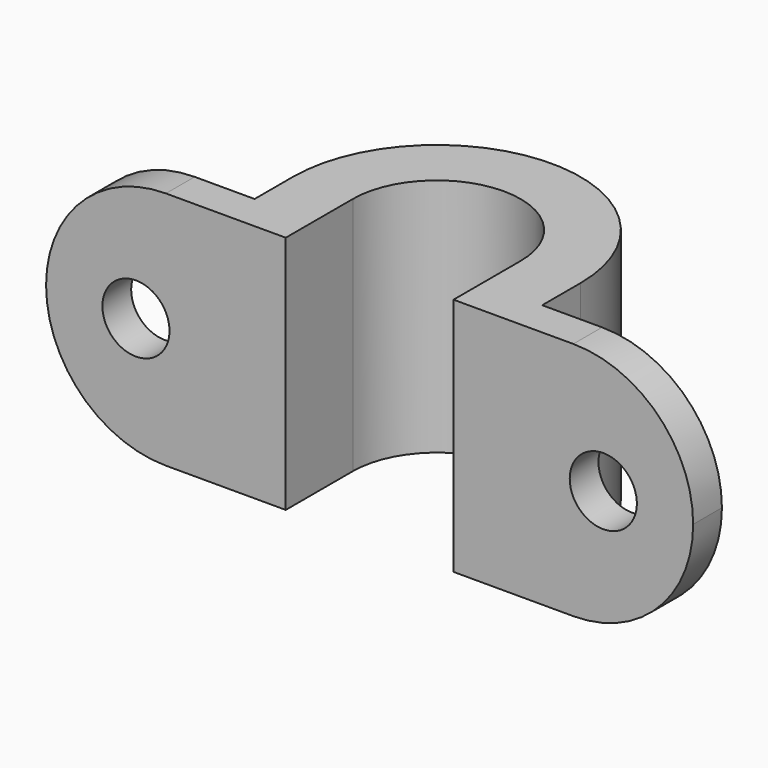
from build123d import *

# Parameters (mm, degrees)
F1_DEPTH = 10
F2_R     = 1.4
F3_DEPTH = 25
F4_R     = 4.99999


# Not quite as in the source:
# - a fillet or chamfer is up to 0.001 mm smaller than in the source, because OpenCascade refuses the exact size


with BuildPart() as f1:
    # F0 (on Top) → F1 (new body)
    with BuildSketch(Plane.XY):
        with BuildLine():
            ThreePointArc((-3.5, 0), (0, 3.5), (3.5, 0))
            Line((3.5, 0), (3.5, -3.5))
            Line((3.5, -3.5), (13.5, -3.5))
            Line((13.5, -3.5), (13.5, -2))
            Line((13.5, -2), (6, -2))
            Line((6, -2), (6, 0))
            ThreePointArc((6, 0), (0, 6), (-6, 0))
            Line((-6, 0), (-6, -2))
            Line((-6, -2), (-13.5, -2))
            Line((-13.5, -2), (-13.5, -3.5))
            Line((-13.5, -3.5), (-3.5, -3.5))
            Line((-3.5, -3.5), (-3.5, 0))
        make_face()
    extrude(amount=F1_DEPTH)

    # F2 (on face) → F3 (cut)
    with BuildSketch(Plane(origin=(0, -2, 0), x_dir=(-1, 0, 0), z_dir=(0, 1, 0))):
        with Locations((9.75, 5)):
            Circle(F2_R)
        with Locations((-9.75, 5)):
            Circle(F2_R)
    extrude(amount=-F3_DEPTH, mode=Mode.SUBTRACT)

    # F4 (radius 5 in the source; OpenCascade refuses exactly that, so slightly less here)
    f4_edges = [f1.edges().sort_by_distance(p)[0] for p in [
        (-13.5, -2.75, 10),
        (13.5, -2.75, 10),
        (-13.5, -2.75, 0),
        (13.5, -2.75, 0),
    ]]
    fillet(f4_edges, radius=F4_R)


solid = f1.part
